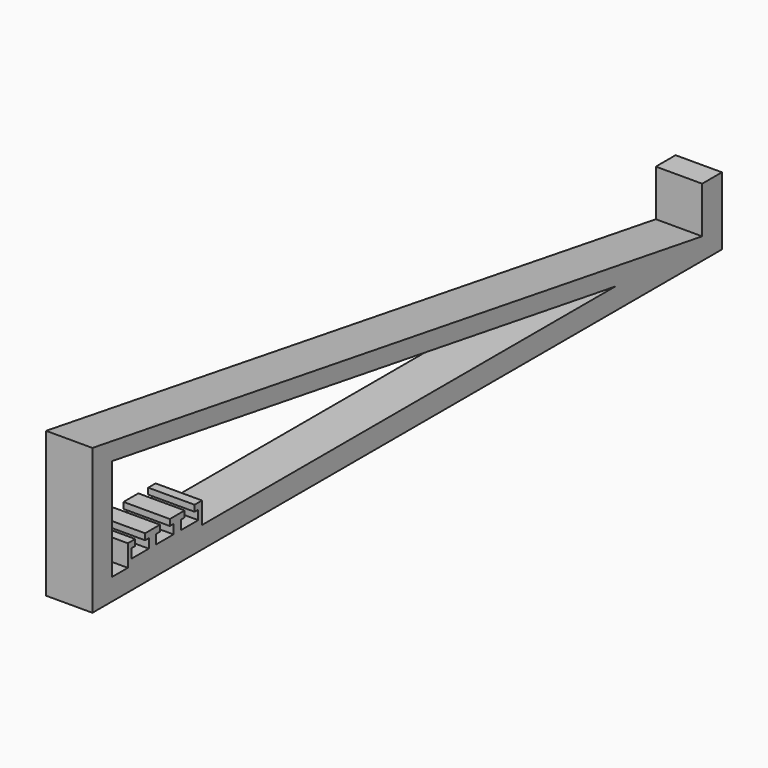
from build123d import *

# Parameters (mm, degrees)
F1_DEPTH = 15


# Not quite as in the source:
# - ends of sketch curves that miss each other by under 0.0002 mm in the source are joined


with BuildPart() as f1:
    # F0 (on Right) → F1 (new body)
    with BuildSketch(Plane.YZ):
        Polygon((73.9477990592, 7), (117.1341684366, 0), (117.1341684366, 22), (109.1341684366, 22), (109.1341684366, 7), align=None)
        Polygon((-129.6450851485, 0), (117.1341684366, 0), (73.9477990592, 7), (-93.3098772168, 7), (-103.3098761737, 7), (-113.3098740876, 7), (-123.3098730445, 7), (-129.6450851485, 7), align=None)
        Polygon((-129.6450851485, 40), (73.9477990592, 7), (109.1341684366, 7), (-137.6450851485, 47), (-137.6450851485, 0), (-129.6450851485, 0), (-129.6450851485, 7), align=None)
        Polygon((-123.3098730445, 14), (-123.3098730445, 7), (-113.3098740876, 7), (-113.3098730445, 14), (-116.3098730445, 14), (-116.3098730445, 12), (-114.8098730445, 12), (-114.8098730445, 9), (-121.8098730445, 9), (-121.8098730445, 12), (-120.3098730445, 12), (-120.3098730445, 14), align=None)
        Polygon((-113.3098740876, 7), (-103.3098761737, 7), (-103.3098751307, 14), (-106.3098751307, 14), (-106.3098751307, 12), (-104.8098751307, 12), (-104.8098751307, 9), (-111.8098751307, 9), (-111.8098751307, 12), (-110.3098751307, 12), (-110.3098751307, 14), (-113.3098751307, 14), align=None)
        Polygon((-103.3098761737, 7), (-93.3098772168, 7), (-93.3098772168, 14), (-96.3098772168, 14), (-96.3098772168, 12), (-94.8098772168, 12), (-94.8098772168, 9), (-101.8098772168, 9), (-101.8098772168, 12), (-100.3098772168, 12), (-100.3098772168, 14), (-103.3098772168, 14), align=None)
    extrude(amount=F1_DEPTH)


solid = f1.part
